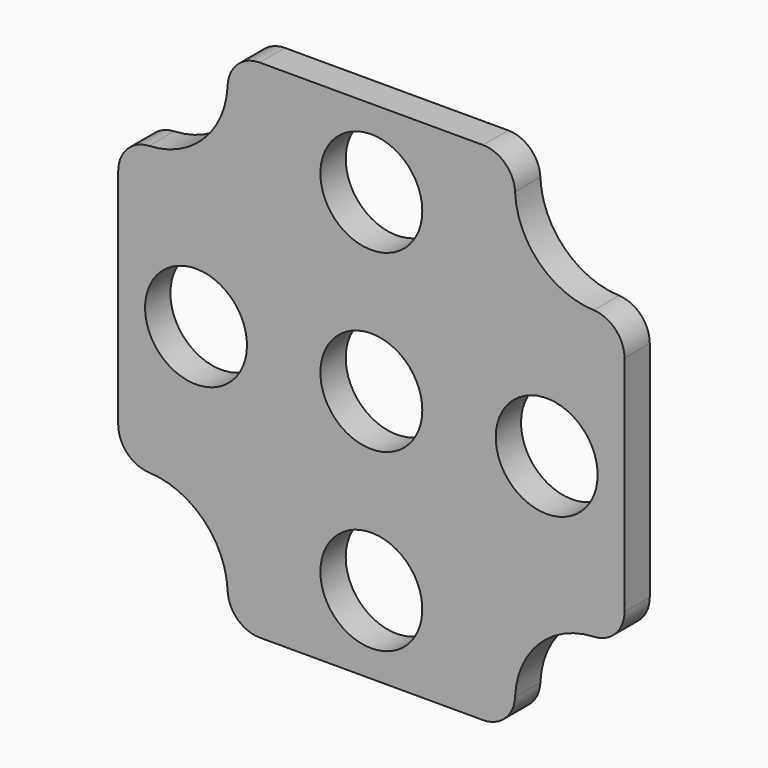
from build123d import *

# Parameters (mm, degrees)
F1_DEPTH        = 5
F4_R            = 8.05
F5_DEPTH        = 5.001
F6_R            = 5.08
F7_R            = 8.05
F8_DEPTH        = 5.001
F8_COPIES_COUNT = 4


# Not quite as in the source:
# - a pattern or mirror of a feature is missing from the dataset's text; its kind, count and spacing are read off the source's solid


with BuildPart() as f1:
    # F0 (on Front) → F1 (new body)
    with BuildSketch(Plane.XZ):
        with BuildLine():
            Line((-40, 23.4314575051), (-40, 0))
            Line((-40, 0), (0, 0))
            Line((0, 0), (0, 40))
            Line((0, 40), (-23.4314575051, 40))
            ThreePointArc((-23.4314575051, 40), (-26.5071641246, 26.5071641246), (-40, 23.4314575051))
        make_face()
    extrude(amount=F1_DEPTH)

    # F2: F1 across face


with BuildPart() as f1_1:
    add(f1.part)
    add(f1.part.mirror(Plane(origin=(0, -2.5, 20), x_dir=(0, 1, 0), z_dir=(1, 0, 0))))

    # F3: F1 across face


with BuildPart() as f1_2:
    add(f1_1.part)
    add(f1_1.part.mirror(Plane(origin=(0, -2.5, 0), x_dir=(1, 0, 0), z_dir=(0, 0, -1))))

    # F4 (on face) → F5 (cut, through all)
    with BuildSketch(Plane.XZ.offset(5)):
        Circle(F4_R)
    extrude(amount=-F5_DEPTH, mode=Mode.SUBTRACT)

    # F6
    f6_edges = [f1_2.edges().sort_by_distance(p)[0] for p in [
        (-40, -2.5, 23.431458),
        (-23.431458, -2.5, 40),
        (23.431458, -2.5, 40),
        (40, -2.5, 23.431458),
        (40, -2.5, -23.431458),
        (23.431458, -2.5, -40),
        (-40, -2.5, -23.431458),
        (-23.431458, -2.5, -40),
    ]]
    fillet(f6_edges, radius=F6_R)

    # F7 (on face) → F8 (cut, through all)
    with BuildSketch(Plane.XZ.offset(5)):
        with Locations((0, 27.7070477605)):
            Circle(F7_R)
    f8 = extrude(amount=-F8_DEPTH, mode=Mode.SUBTRACT)

    # F8_copies: F8 ×4 about axis
    f8_copies_axis = Axis((0, 0, 0), (0, 1, 0))
    for i in range(1, F8_COPIES_COUNT):
        add(f8.rotate(f8_copies_axis, i * 360 / F8_COPIES_COUNT), mode=Mode.SUBTRACT)


solid = f1_2.part
